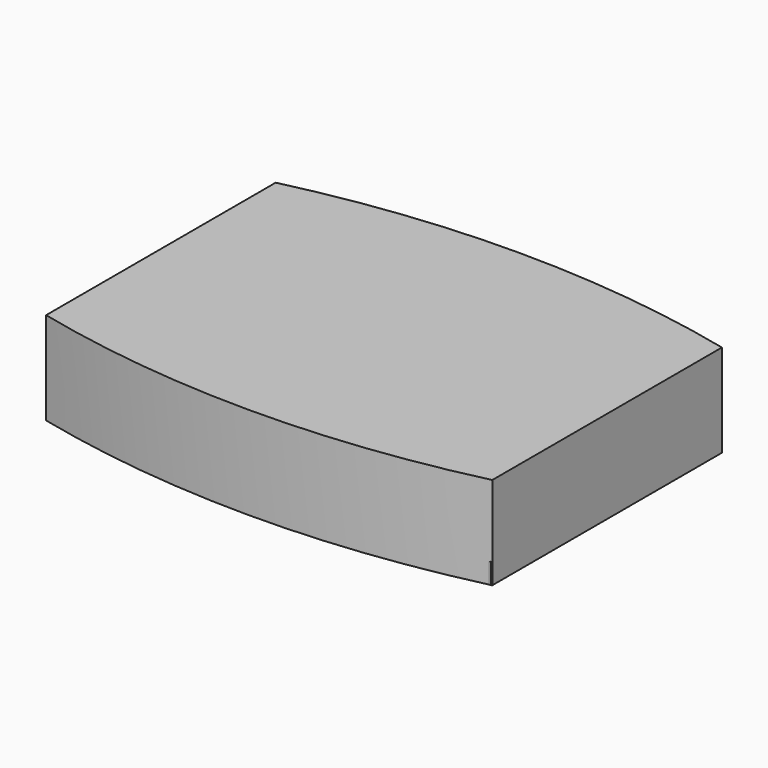
from build123d import *

# Parameters (mm, degrees)
F0_W     = 122.2604140639
F0_H     = 78.6352567375
F2_DEPTH = 25.4
F3_T     = -2.54
F1_W     = 63.6047422886
F1_H     = 78.8185559213
F4_DEPTH = 5.588
F5_R     = 1.6394762834
F6_DEPTH = 28.194
F5_R_2   = 1.6394765438
F7_DEPTH = 32.258


# Not quite as in the source:
# - the program builds the solid bodies; features that only make, move or delete a surface that nothing else refers to are left out


with BuildPart() as f2:
    # F0 (on Top) → F2 (new body)
    with BuildSketch(Plane.XY):
        with BuildLine():
            ThreePointArc((63.7880414724, 35.6516502798), (2.6578344405, 42.8155765092), (-58.4723725915, 35.6516502798))
            Line((-58.4723725915, 35.6516502798), (63.7880414724, 35.6516502798))
        make_face()
        with Locations((2.6578344405, -3.665978089)):
            Rectangle(F0_W, F0_H)
        with BuildLine():
            Line((63.7880414724, -42.9836064577), (-58.4723725915, -42.9836064577))
            ThreePointArc((-58.4723725915, -42.9836064577), (2.6578344405, -50.1645132958), (63.7880414724, -42.9836064577))
        make_face()
    extrude(amount=F2_DEPTH)

    # F3
    f3_openings = [f2.faces().sort_by_distance(p)[0] for p in [
        (-58.472373, -3.665978, 12.7),
    ]]
    offset(amount=F3_T, openings=f3_openings)

    # F1 (on Top) → F4 (join)
    with BuildSketch(Plane.XY):
        with Locations((31.8023711443, -3.7576276809)):
            Rectangle(F1_W, F1_H)
    extrude(amount=F4_DEPTH)

    # F5 (on Front) → F6 (cut)
    with BuildSketch(Plane.XZ):
        with Locations((-47.8410311043, 4.857422784)):
            Circle(F5_R)
    extrude(amount=-F6_DEPTH, mode=Mode.SUBTRACT)

    # F5 (on Front) → F7 (cut)
    with BuildSketch(Plane.XZ):
        with Locations((-13.1975244731, 4.857422784)):
            Circle(F5_R_2)
        with Locations((-47.8410311043, 4.857422784)):
            Circle(F5_R)
    extrude(amount=-F7_DEPTH, mode=Mode.SUBTRACT)


solid = f2.part
